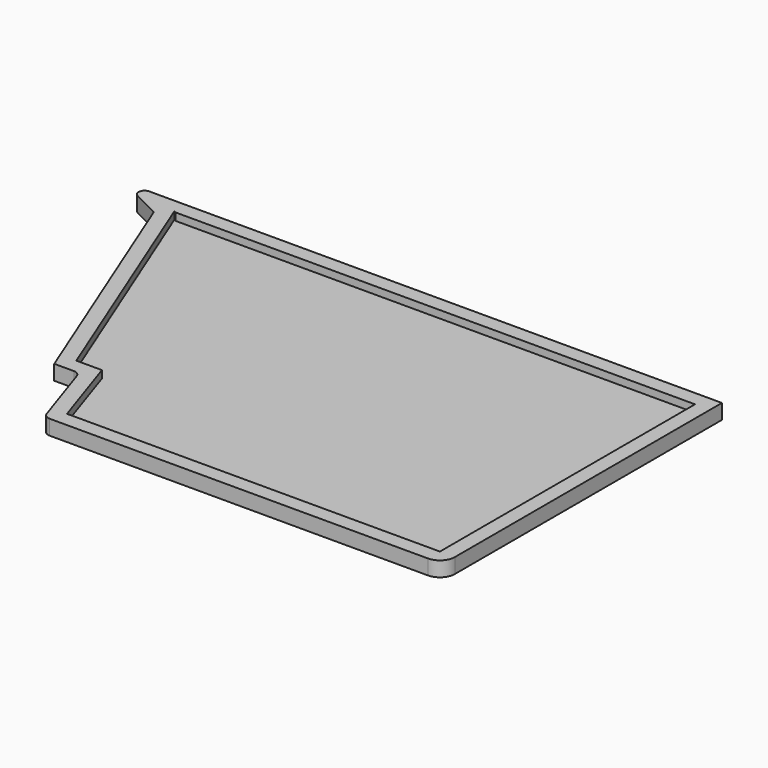
from build123d import *

# Parameters (mm, degrees)
F1_DEPTH    = 1.5
F2_DEPTH    = 1.5
F3_T1_DEPTH = 28.416407865
F4_R        = 1.25
F5_R        = 1.5
F6_R        = 3


# Not quite as in the source:
# - a fillet or chamfer that OpenCascade refuses, or shapes differently, is made with other operations: its cross-section is extruded or revolved along the edge and cut away or added
# - a feature names something its author has since deleted; it is built from what else it names


with BuildPart() as f1:
    # F0 (on Top) → F1 (new body)
    with BuildSketch(Plane.XY):
        Polygon((40, -35), (40, 35), (-40, 35), (-80, 35), (-70, 30), (-50, -20), (-45, -20), (-40, -35), align=None)
        Polygon((-37.8377223398, -32), (-42.8377223398, -17), (-47.9689011157, -17), (-67.6381773778, 32.1731906551), (-67.2917960675, 32), (-40, 32), (37, 32), (37, -32), align=None, mode=Mode.SUBTRACT)
        Polygon((-47.9689011157, -17), (-42.8377223398, -17), (-37.8377223398, -32), (37, -32), (37, 32), (-40, 32), (-67.2917960675, 32), (-67.6381773778, 32.1731906551), align=None)
    extrude(amount=-F1_DEPTH)

    # F0 (on Top) → F2 (join)
    with BuildSketch(Plane.XY):
        Polygon((40, -35), (40, 35), (-40, 35), (-80, 35), (-70, 30), (-50, -20), (-45, -20), (-40, -35), align=None)
        Polygon((-37.8377223398, -32), (-42.8377223398, -17), (-47.9689011157, -17), (-67.6381773778, 32.1731906551), (-67.2917960675, 32), (-40, 32), (37, 32), (37, -32), align=None, mode=Mode.SUBTRACT)
    extrude(amount=F2_DEPTH)

    # F3: fillet of radius 1.2 on 1 edges, made by hand

    # F3_s2 → F3_t1 (cut)
    with BuildSketch(Plane.XY.offset(-14.2082039325)):
        with BuildLine():
            ThreePointArc((-75.4533747416, 32.7266873708), (-76.0846172144, 34.0757035047), (-74.916718427, 35))
            Line((-74.916718427, 35), (-80, 35))
            Line((-80, 35), (-75.4533747416, 32.7266873708))
        make_face()
    extrude(amount=F3_T1_DEPTH, mode=Mode.SUBTRACT)

    # F4
    f4_edges = [f1.edges().sort_by_distance(p)[0] for p in [
        (-70, 30, 0),
    ]]
    fillet(f4_edges, radius=F4_R)

    # F5
    f5_edges = [f1.edges().sort_by_distance(p)[0] for p in [
        (-45, -20, 0),
        (-40, -35, 0),
    ]]
    fillet(f5_edges, radius=F5_R)

    # F6
    f6_edges = [f1.edges().sort_by_distance(p)[0] for p in [
        (40, -35, 0),
    ]]
    fillet(f6_edges, radius=F6_R)


solid = f1.part
